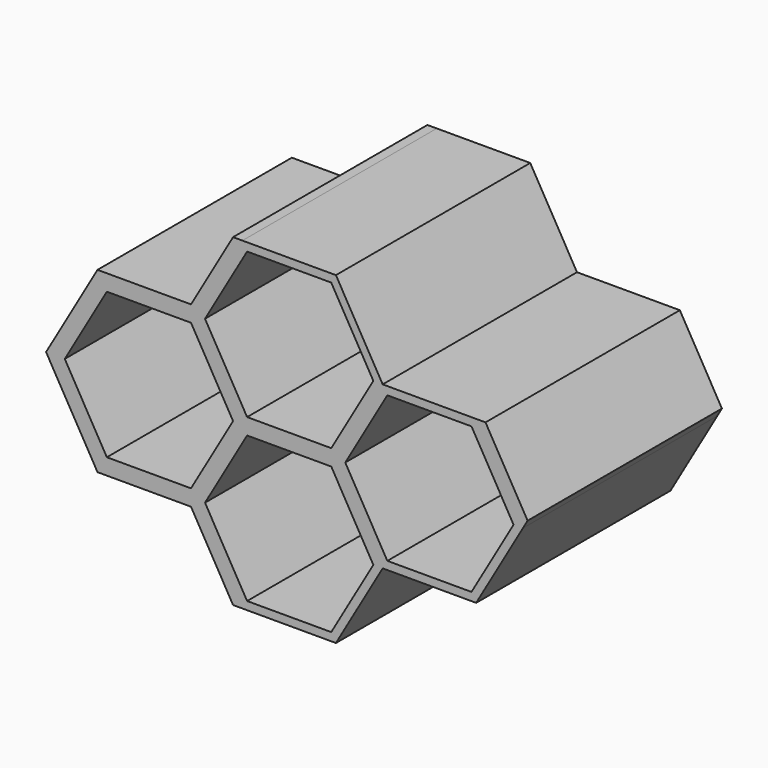
from build123d import *

# Parameters (mm, degrees)
F1_DEPTH = 12.7
F2_DEPTH = 95.25


# Not quite as in the source:
# - a feature names something its author has since deleted; it is built from what else it names


with BuildPart() as f1:
    # F0 (on Front) → F1 (new body)
    with BuildSketch(Plane.XZ):
        Polygon((-132.5943648094, 3.2924993012), (-114.2634937626, 35.0424993012), (-132.5943648094, 66.7924993012), (-169.2561069029, 66.7924993012), (-187.5869779497, 35.0424993012), (-169.2561069029, 3.2924993012), align=None)
        Polygon((-167.4230197982, 6.4674993012), (-183.9208037403, 35.0424993012), (-167.4230197982, 63.6174993012), (-134.427451914, 63.6174993012), (-117.929667972, 35.0424993012), (-134.427451914, 6.4674993012), align=None, mode=Mode.SUBTRACT)
        Polygon((-114.2634937626, 35.0424993012), (-77.6017516691, 35.0424993012), (-59.2708806223, 66.7924993012), (-77.6017516691, 98.5424993012), (-114.2634937626, 98.5424993012), (-132.5943648094, 66.7924993012), align=None)
        Polygon((-112.4304066579, 38.2174993012), (-128.9281906, 66.7924993012), (-112.4304066579, 95.3674993012), (-79.4348387737, 95.3674993012), (-62.9370548316, 66.7924993012), (-79.4348387737, 38.2174993012), align=None, mode=Mode.SUBTRACT)
        Polygon((-169.2561069029, 66.7924993012), (-132.5943648094, 66.7924993012), (-114.2634937626, 98.5424993012), (-132.5943648094, 130.2924993012), (-169.2561069029, 130.2924993012), (-187.5869779497, 98.5424993012), align=None)
        Polygon((-167.4230197982, 69.9674993012), (-183.9208037403, 98.5424993012), (-167.4230197982, 127.1174993012), (-134.427451914, 127.1174993012), (-117.929667972, 98.5424993012), (-134.427451914, 69.9674993012), align=None, mode=Mode.SUBTRACT)
        Polygon((-187.5869779497, 35.0424993012), (-169.2561069029, 66.7924993012), (-187.5869779497, 98.5424993012), (-190.6410588775, 98.5424993012), (-224.2487200432, 98.5424993012), (-242.57959109, 66.7924993012), (-224.2487200432, 35.0424993012), (-221.8035396555, 35.0424993012), align=None)
        Polygon((-222.4156329385, 38.2174993012), (-238.9134168806, 66.7924993012), (-222.4156329385, 95.3674993012), (-189.4200650544, 95.3674993012), (-172.9222811123, 66.7924993012), (-189.4200650544, 38.2174993012), align=None, mode=Mode.SUBTRACT)
        Polygon((-222.4156329385, 95.3674993012), (-238.9134168806, 66.7924993012), (-222.4156329385, 38.2174993012), (-189.4200650544, 38.2174993012), (-172.9222811123, 66.7924993012), (-189.4200650544, 95.3674993012), align=None)
        Polygon((-167.4230197982, 127.1174993012), (-183.9208037403, 98.5424993012), (-167.4230197982, 69.9674993012), (-134.427451914, 69.9674993012), (-117.929667972, 98.5424993012), (-134.427451914, 127.1174993012), align=None)
        Polygon((-167.4230197982, 63.6174993012), (-183.9208037403, 35.0424993012), (-167.4230197982, 6.4674993012), (-134.427451914, 6.4674993012), (-117.929667972, 35.0424993012), (-134.427451914, 63.6174993012), align=None)
        Polygon((-112.4304066579, 95.3674993012), (-128.9281906, 66.7924993012), (-112.4304066579, 38.2174993012), (-79.4348387737, 38.2174993012), (-62.9370548316, 66.7924993012), (-79.4348387737, 95.3674993012), align=None)
    extrude(amount=F1_DEPTH)

    # F0 (on Front) → F2 (join)
    with BuildSketch(Plane.XZ):
        Polygon((-114.2634937626, 35.0424993012), (-77.6017516691, 35.0424993012), (-59.2708806223, 66.7924993012), (-77.6017516691, 98.5424993012), (-114.2634937626, 98.5424993012), (-132.5943648094, 66.7924993012), align=None)
        Polygon((-112.4304066579, 38.2174993012), (-128.9281906, 66.7924993012), (-112.4304066579, 95.3674993012), (-79.4348387737, 95.3674993012), (-62.9370548316, 66.7924993012), (-79.4348387737, 38.2174993012), align=None, mode=Mode.SUBTRACT)
        Polygon((-77.6017516691, 98.5424993012), (-59.2708806223, 66.7924993012), (-57.4377935176, 69.9674993012), (-73.9355774597, 98.5424993012), align=None)
        Polygon((-132.5943648094, 3.2924993012), (-114.2634937626, 35.0424993012), (-132.5943648094, 66.7924993012), (-169.2561069029, 66.7924993012), (-187.5869779497, 35.0424993012), (-169.2561069029, 3.2924993012), align=None)
        Polygon((-167.4230197982, 6.4674993012), (-183.9208037403, 35.0424993012), (-167.4230197982, 63.6174993012), (-134.427451914, 63.6174993012), (-117.929667972, 35.0424993012), (-134.427451914, 6.4674993012), align=None, mode=Mode.SUBTRACT)
        Polygon((-169.2561069029, 66.7924993012), (-132.5943648094, 66.7924993012), (-114.2634937626, 98.5424993012), (-132.5943648094, 130.2924993012), (-169.2561069029, 130.2924993012), (-187.5869779497, 98.5424993012), align=None)
        Polygon((-167.4230197982, 69.9674993012), (-183.9208037403, 98.5424993012), (-167.4230197982, 127.1174993012), (-134.427451914, 127.1174993012), (-117.929667972, 98.5424993012), (-134.427451914, 69.9674993012), align=None, mode=Mode.SUBTRACT)
        Polygon((-172.9222811123, 3.2924993012), (-169.2561069029, 3.2924993012), (-187.5869779497, 35.0424993012), (-221.8035396555, 35.0424993012), (-224.2487200432, 35.0424993012), (-242.57959109, 66.7924993012), (-224.2487200432, 98.5424993012), (-190.6410588775, 98.5424993012), (-187.5869779497, 98.5424993012), (-169.2561069029, 130.2924993012), (-172.9222811123, 130.2924993011), (-189.4200650544, 101.7174993012), (-226.0818071479, 101.7174993012), (-246.2457652993, 66.7924993012), (-226.0818071479, 31.8674993012), (-189.4200650544, 31.8674993012), align=None)
        Polygon((-187.5869779497, 35.0424993012), (-169.2561069029, 66.7924993012), (-187.5869779497, 98.5424993012), (-190.6410588775, 98.5424993012), (-224.2487200432, 98.5424993012), (-242.57959109, 66.7924993012), (-224.2487200432, 35.0424993012), (-221.8035396555, 35.0424993012), align=None)
        Polygon((-222.4156329385, 38.2174993012), (-238.9134168806, 66.7924993012), (-222.4156329385, 95.3674993012), (-189.4200650544, 95.3674993012), (-172.9222811123, 66.7924993012), (-189.4200650544, 38.2174993012), align=None, mode=Mode.SUBTRACT)
    extrude(amount=F2_DEPTH)


solid = f1.part
